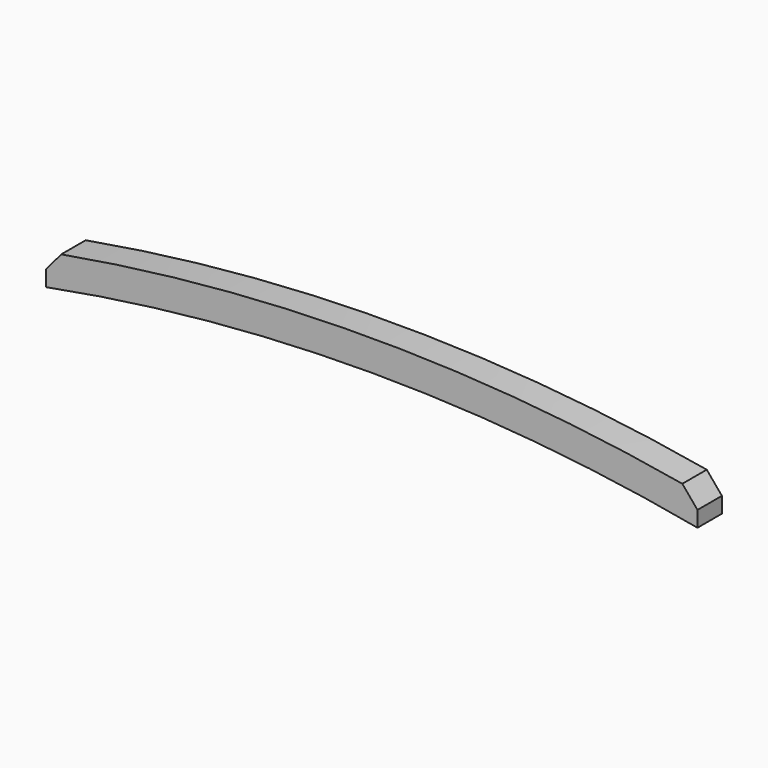
from build123d import *

# Parameters (mm, degrees)
F1_DEPTH    = 19.05
F2_T1_DEPTH = 68.6123794065


# Not quite as in the source:
# - a fillet or chamfer that OpenCascade refuses, or shapes differently, is made with other operations: its cross-section is extruded or revolved along the edge and cut away or added


with BuildPart() as f1:
    # F0 (on Front) → F1 (new body)
    with BuildSketch(Plane.XZ):
        with BuildLine():
            ThreePointArc((-203.2046722501, -19.05), (0, 0), (203.2046722501, -19.05))
            Line((203.2046722501, -19.05), (203.2046722501, 0.3318805247))
            ThreePointArc((203.2046722501, 0.3318805247), (0, 19.0500002354), (-203.2046722501, 0.3318805247))
            Line((-203.2046722501, 0.3318805247), (-203.2046722501, -19.05))
        make_face()
    extrude(amount=F1_DEPTH)

    # F2: chamfer of 9.525 on 2 edges, made by hand

    # F2_s2 → F2_t1 (cut)
    with BuildSketch(Plane.XZ.offset(-24.7811897032)):
        with BuildLine():
            Line((-193.4976640556, 2.339657905), (-203.4494965837, -9.5268916064))
            Line((-203.4494965837, -9.5268916064), (-203.6399965837, -9.5268916064))
            ThreePointArc((-203.6399965837, -9.5268916064), (-203.3951722501, -4.5975055408), (-203.3951722501, 0.3318805247))
            Line((-203.3951722501, 0.3318805247), (-203.2394726328, 0.5191749009))
            ThreePointArc((-203.2394726328, 0.5191749009), (-198.3652719444, 1.4136040473), (-193.5308439656, 2.5272461338))
            Line((-193.5308439656, 2.5272461338), (-193.4976640556, 2.339657905))
        make_face()
        with BuildLine():
            Line((193.4976640556, 2.339657905), (203.4494965837, -9.5268916064))
            Line((203.4494965837, -9.5268916064), (203.6399965837, -9.5268916064))
            ThreePointArc((203.6399965837, -9.5268916064), (203.3951722501, -4.5975055408), (203.3951722501, 0.3318805247))
            Line((203.3951722501, 0.3318805247), (203.2394726328, 0.5191749009))
            ThreePointArc((203.2394726328, 0.5191749009), (198.3652719444, 1.4136040473), (193.5308439656, 2.5272461338))
            Line((193.5308439656, 2.5272461338), (193.4976640556, 2.339657905))
        make_face()
    extrude(amount=F2_T1_DEPTH, mode=Mode.SUBTRACT)


solid = f1.part
